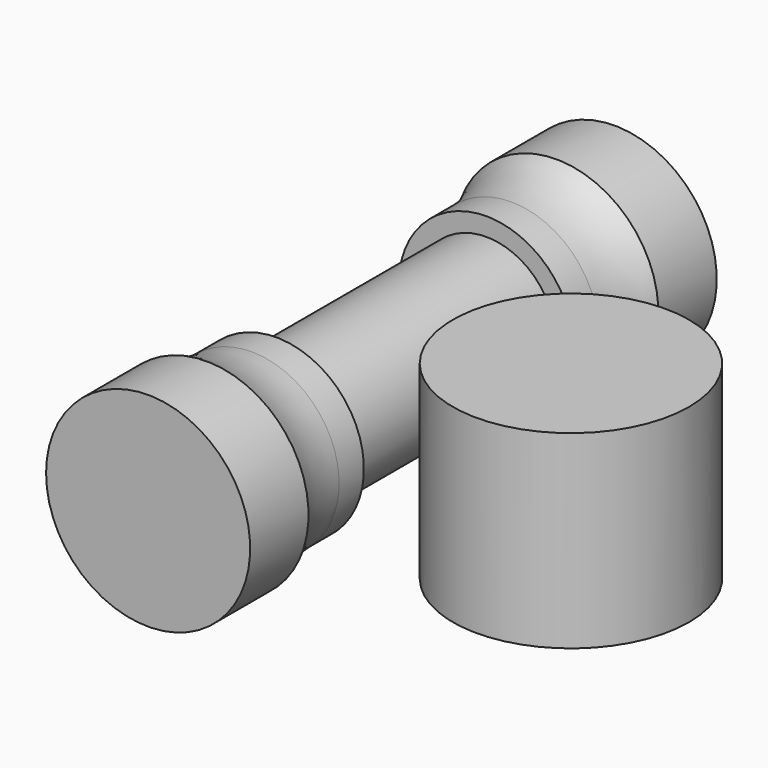
from build123d import *

# Parameters (mm, degrees)
F4_R     = 8.1
F5_DEPTH = 13


# Not quite as in the source:
# - a fillet or chamfer that OpenCascade refuses, or shapes differently, is made with other operations: its cross-section is extruded or revolved along the edge and cut away or added


with BuildPart() as f3:
    # F2 (on offset) → F3 (revolve)
    with BuildSketch(Plane.XY.offset(8)):
        Polygon((-20, 15), (-19, 15), (-19, 9), (-17.75, 9), (-17.75, -9), (-19, -9), (-19, -15), (-20, -15), (-20, -20), (-13, -20), (-13, 20), (-20, 20), align=None)
    revolve(axis=Axis((-13, 1.0613519698, 8), (0, -1, 0)))

    # F6: fillet of radius 8 on 2 edges, made by hand

    # F6_s1 → F6_t2 (revolve)
    with BuildSketch(Plane.XY.offset(8)):
        with BuildLine():
            ThreePointArc((-20, 15), (-19.2540333076, 13.1270166538), (-19, 11.1270166538))
            Line((-19, 11.1270166538), (-19, 15))
            Line((-19, 15), (-20, 15))
        make_face()
    revolve(axis=Axis((-13, 15, 8), (0, -1, 0)))

    # F6_s3 → F6_t4 (revolve)
    with BuildSketch(Plane.XY.offset(8)):
        with BuildLine():
            ThreePointArc((-19, -11.1270166538), (-19.2540333076, -13.1270166538), (-20, -15))
            Line((-20, -15), (-19, -15))
            Line((-19, -15), (-19, -11.1270166538))
        make_face()
    revolve(axis=Axis((-13, -15, 8), (0, -1, 0)))


with BuildPart() as f5:
    # F4 (on Top) → F5 (new body)
    with BuildSketch(Plane.XY):
        Circle(F4_R)
    extrude(amount=F5_DEPTH)


solid = Compound([f3.part, f5.part])
